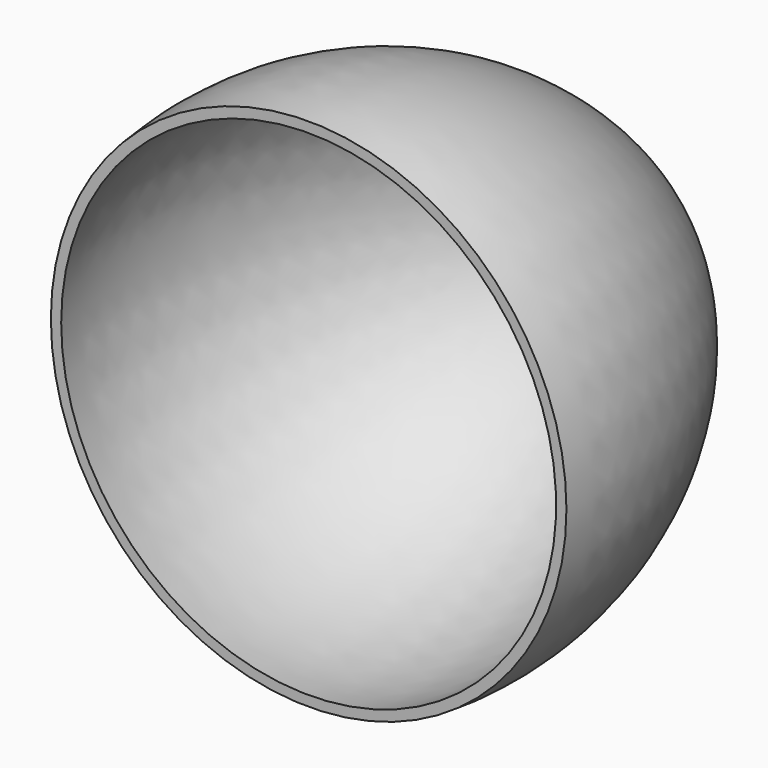
from build123d import *


# Not quite as in the source:
# - a feature names something its author has since deleted; it is built from what else it names


with BuildPart() as f1:
    # F0 (on Top) → F1 (revolve)
    with BuildSketch(Plane.XY):
        with BuildLine():
            ThreePointArc((0, 40), (-19.6969266743, 24.4980791714), (-25, 0))
            Line((-25, 0), (-24, 0))
            ThreePointArc((-24, 0), (-19.2876490579, 23.9847071126), (0, 39))
            Line((0, 39), (0, 40))
        make_face()
    revolve(axis=Axis((0, 19.5, 0), (0, -1, 0)))


solid = f1.part
